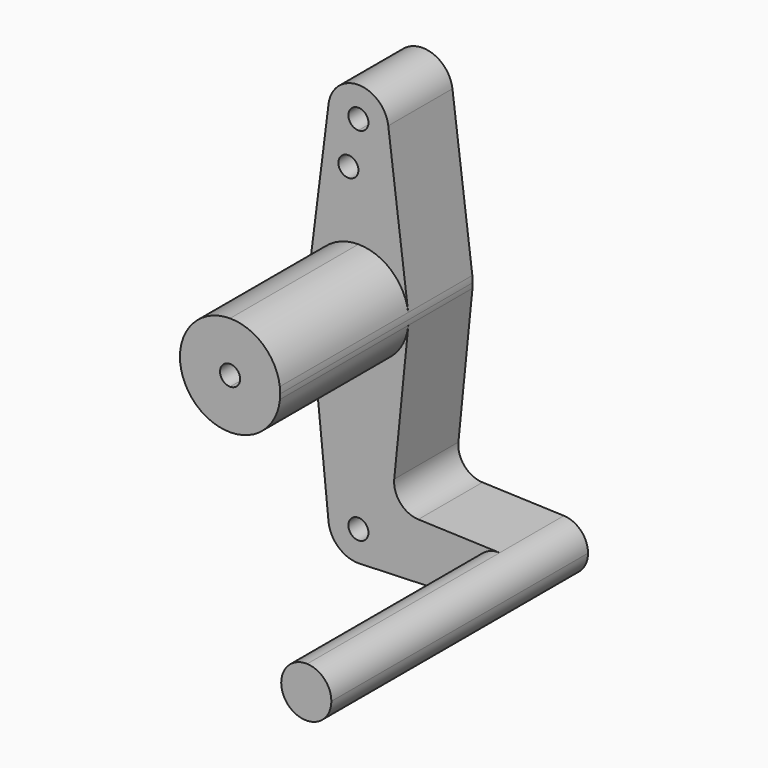
from build123d import *

# Parameters (mm, degrees)
F1_DEPTH = 1
F0_R     = 0.125
F2_DEPTH = 3
F3_DEPTH = 4


with BuildPart() as f1:
    # F0 (on Front) → F1 (new body)
    with BuildSketch(Plane.XZ):
        with BuildLine():
            Line((1.4375, 0), (0.375, 0))
            ThreePointArc((0.375, 0), (0.2698585939, -0.2603869031), (0.0133928571, -0.3747607655))
            Line((0.0133928571, -0.3747607655), (1.7611607143, -0.3123006379))
            ThreePointArc((1.7611607143, -0.3123006379), (1.5330109141, -0.2248821616), (1.4375, 0))
        make_face()
        with BuildLine():
            Line((0.375, 0), (0.125, 0))
            ThreePointArc((0.125, 0), (-0.0883883476, -0.0883883476), (0, 0.125))
            Line((0, 0.125), (0, 0.375))
            ThreePointArc((0, 0.375), (-0.2781074433, 0.2515576475), (-0.3731202889, -0.0375))
            ThreePointArc((-0.3731202889, -0.0375), (-0.2465505268, -0.2825559019), (0.0133928571, -0.3747607655))
            ThreePointArc((0.0133928571, -0.3747607655), (0.2698585939, -0.2603869031), (0.375, 0))
        make_face()
        with BuildLine():
            ThreePointArc((0, 0.375), (0.2651650429, 0.2651650429), (0.375, 0))
            Line((0.375, 0), (1.4375, 0))
            ThreePointArc((1.4375, 0), (1.5330109141, 0.2248821616), (1.7611607143, 0.3123006379))
            Line((1.7611607143, 0.3123006379), (0.7467559055, 0.3485525083))
            ThreePointArc((0.7467559055, 0.3485525083), (0.5220944841, 0.4555653209), (0.4465034091, 0.6926528273))
            Line((0.4465034091, 0.6926528273), (0.6218671482, 2.4375))
            ThreePointArc((0.6218671482, 2.4375), (0.4192627458, 2.0364875946), (0, 1.875))
            Line((0, 1.875), (0, 0.375))
        make_face()
        with BuildLine():
            ThreePointArc((-0.3731202889, -0.0375), (-0.2781074433, 0.2515576475), (0, 0.375))
            Line((0, 0.375), (0, 1.875))
            ThreePointArc((0, 1.875), (-0.4192627458, 2.0364875946), (-0.6218671482, 2.4375))
            Line((-0.6218671482, 2.4375), (-0.3731202889, -0.0375))
        make_face()
        with BuildLine():
            ThreePointArc((0, 0.125), (0.0883883476, 0.0883883476), (0.125, 0))
            Line((0.125, 0), (0.375, 0))
            ThreePointArc((0.375, 0), (0.2651650429, 0.2651650429), (0, 0.375))
            Line((0, 0.375), (0, 0.125))
        make_face()
    extrude(amount=F1_DEPTH)

    # F0 (on Front) → F3 (join)
    with BuildSketch(Plane.XZ):
        with BuildLine():
            ThreePointArc((1.7611607143, 0.3123006379), (1.5330109141, 0.2248821616), (1.4375, 0))
            ThreePointArc((1.4375, 0), (1.5330109141, -0.2248821616), (1.7611607143, -0.3123006379))
            ThreePointArc((1.7611607143, -0.3123006379), (1.9748821616, -0.2169890859), (2.0625, 0))
            ThreePointArc((2.0625, 0), (1.9748821616, 0.2169890859), (1.7611607143, 0.3123006379))
        make_face()
        with BuildLine():
            ThreePointArc((1.875, 0), (1.75, -0.125), (1.625, 0))
            ThreePointArc((1.625, 0), (1.75, 0.125), (1.875, 0))
        make_face(mode=Mode.SUBTRACT)
        with BuildLine():
            ThreePointArc((1.875, 0), (1.75, 0.125), (1.625, 0))
            ThreePointArc((1.625, 0), (1.75, -0.125), (1.875, 0))
        make_face()
    extrude(amount=F3_DEPTH)


with BuildPart() as f1b:
    # F0 (on Front) → F1, piece 2 (new body)
    with BuildSketch(Plane.XZ):
        with BuildLine():
            Line((0, 3.938), (0, 3.125))
            ThreePointArc((0, 3.125), (0.4133986424, 2.96875), (0.6200979635, 2.578125))
            Line((0.6200979635, 2.578125), (0.3720587781, 4.546875))
            ThreePointArc((0.3720587781, 4.546875), (0.3742639722, 4.5234835922), (0.375, 4.5))
            ThreePointArc((0.375, 4.5), (0.2651650429, 4.2348349571), (0, 4.125))
            Line((0, 4.125), (0, 3.938))
        make_face()
        with BuildLine():
            Line((-0.3720587781, 4.546875), (-0.6200979635, 2.578125))
            ThreePointArc((-0.6200979635, 2.578125), (-0.4133986424, 2.96875), (0, 3.125))
            Line((0, 3.125), (0, 3.938))
            Line((0, 3.938), (0, 4.125))
            ThreePointArc((0, 4.125), (-0.28125, 4.2519608146), (-0.3720587781, 4.546875))
        make_face()
        with Locations((-0.125, 3.938)):
            Circle(F0_R, mode=Mode.SUBTRACT)
        with BuildLine():
            ThreePointArc((0.3720587781, 4.546875), (0, 4.875), (-0.3720587781, 4.546875))
            ThreePointArc((-0.3720587781, 4.546875), (-0.28125, 4.2519608146), (0, 4.125))
            ThreePointArc((0, 4.125), (0.2651650429, 4.2348349571), (0.375, 4.5))
            ThreePointArc((0.375, 4.5), (0.3742639722, 4.5234835922), (0.3720587781, 4.546875))
        make_face()
        with BuildLine():
            ThreePointArc((0.125, 4.5), (0.0883883476, 4.4116116524), (0, 4.375))
            ThreePointArc((0, 4.375), (-0.0883883476, 4.5883883476), (0.125, 4.5))
        make_face(mode=Mode.SUBTRACT)
    extrude(amount=F1_DEPTH)


with BuildPart() as f2:
    # F0 (on Front) → F2 (new body)
    with BuildSketch(Plane.XZ):
        with BuildLine():
            Line((0, 2.375), (0, 1.875))
            ThreePointArc((0, 1.875), (0.4192627458, 2.0364875946), (0.6218671482, 2.4375))
            ThreePointArc((0.6218671482, 2.4375), (0.6242162957, 2.4687107656), (0.625, 2.5))
            ThreePointArc((0.625, 2.5), (0.623773287, 2.5391393203), (0.6200979635, 2.578125))
            ThreePointArc((0.6200979635, 2.578125), (0.4133986424, 2.96875), (0, 3.125))
            Line((0, 3.125), (0, 2.625))
            ThreePointArc((0, 2.625), (0.0883883476, 2.5883883476), (0.125, 2.5))
            ThreePointArc((0.125, 2.5), (0.0883883476, 2.4116116524), (0, 2.375))
        make_face()
        with BuildLine():
            ThreePointArc((-0.6218671482, 2.4375), (-0.4192627458, 2.0364875946), (0, 1.875))
            Line((0, 1.875), (0, 2.375))
            ThreePointArc((0, 2.375), (-0.125, 2.5), (0, 2.625))
            Line((0, 2.625), (0, 3.125))
            ThreePointArc((0, 3.125), (-0.4133986424, 2.96875), (-0.6200979635, 2.578125))
            ThreePointArc((-0.6200979635, 2.578125), (-0.6249505439, 2.5078624207), (-0.6218671482, 2.4375))
        make_face()
    extrude(amount=F2_DEPTH)


solid = Compound([f1.part, f1b.part, f2.part])
